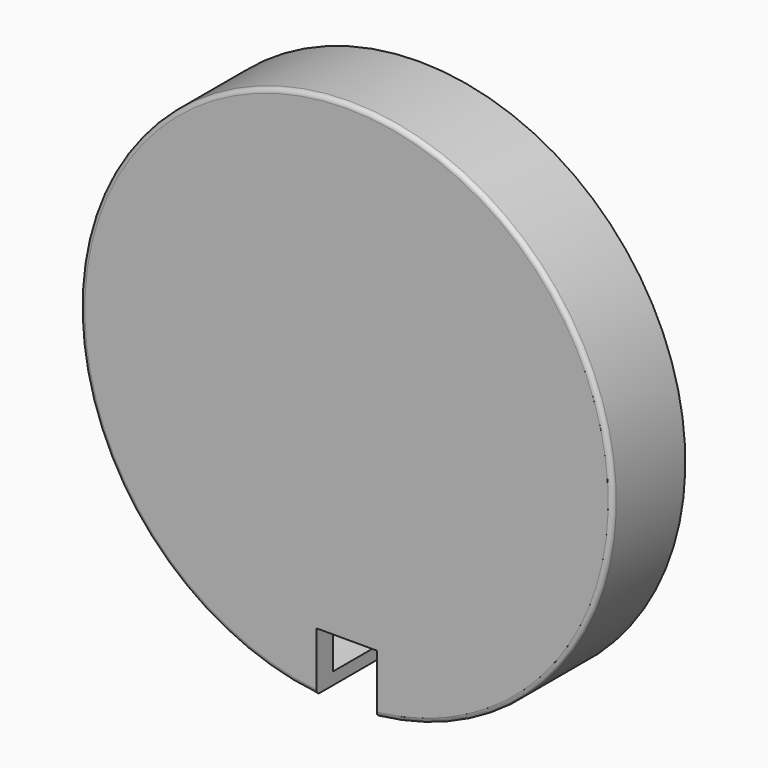
from build123d import *

# Parameters (mm, degrees)
F0_R     = 88
F1_DEPTH = 30
F2_R     = 84
F3_DEPTH = 23
F4_R     = 1.5
F5_W     = 20
F5_H     = 20
F6_DEPTH = 30.001


# Not quite as in the source:
# - a feature names something its author has since deleted; it is built from what else it names


with BuildPart() as f1:
    # F0 (on Front) → F1 (new body)
    with BuildSketch(Plane.XZ):
        Circle(F0_R)
    extrude(amount=F1_DEPTH)

    # F2 (on face) → F3 (cut)
    with BuildSketch(Plane(origin=(0, 0, 0), x_dir=(-1, 0, 0), z_dir=(0, 1, 0))):
        Circle(F2_R)
    extrude(amount=-F3_DEPTH, mode=Mode.SUBTRACT)

    # F4
    f4_edges = [f1.edges().sort_by_distance(p)[0] for p in [
        (-88, -30, 0),
    ]]
    fillet(f4_edges, radius=F4_R)

    # F5 (on face) → F6 (cut, through all)
    with BuildSketch(Plane.XZ.offset(30)):
        with Locations((0, -78)):
            Rectangle(F5_W, F5_H)
    extrude(amount=-F6_DEPTH, mode=Mode.SUBTRACT)


solid = f1.part
